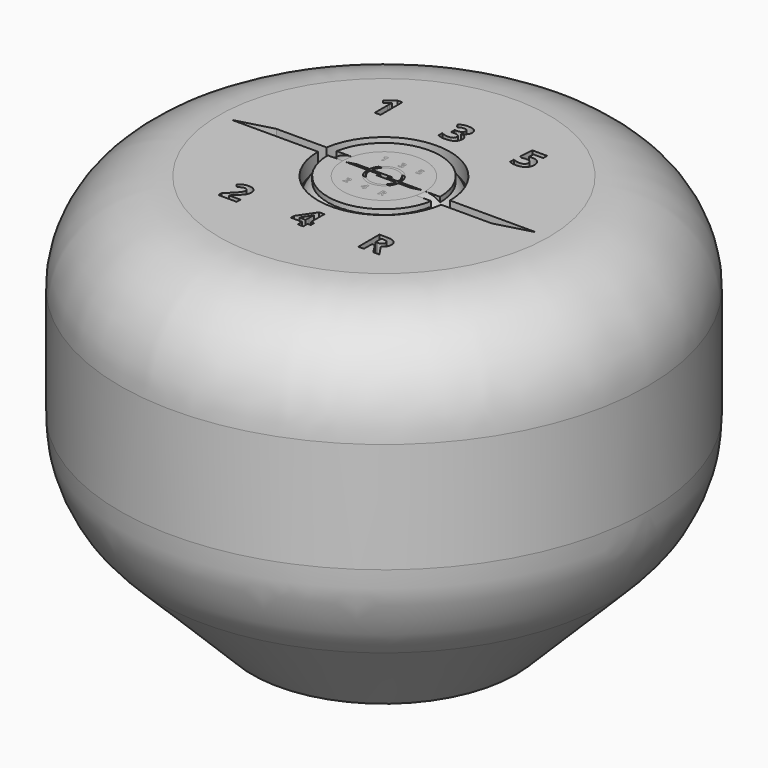
from build123d import *

# Parameters (mm, degrees)
F1_R           = 101.6
F2_DEPTH       = 152.4
F3_R           = 38.1
F4_SIZE        = 50.8
F5_R           = 50.8
F6_TEXT_SIZE   = 14.6624815095
F6_TEXT_SIZE_2 = 14.2217245241
F7_DEPTH       = 6.35
F8_SCALE       = 0.25


# Not quite as in the source:
# - Text() gives the source's letters only with a copy of the font that has no kerning and outlines rounded to 1/6400 em; it was checked with that copy


with BuildPart() as f2:
    # F1 (on Top) → F2 (new body)
    with BuildSketch(Plane.XY):
        Circle(F1_R)
    extrude(amount=-F2_DEPTH)

    # F3
    f3_edges = [f2.edges().sort_by_distance(p)[0] for p in [
        (-101.6, 0, 0),
    ]]
    fillet(f3_edges, radius=F3_R)

    # F4
    f4_edges = [f2.edges().sort_by_distance(p)[0] for p in [
        (-101.6, 0, -152.4),
    ]]
    chamfer(f4_edges, length=F4_SIZE)

    # F5
    f5_edges = [f2.edges().sort_by_distance(p)[0] for p in [
        (-101.6, 0, -101.6),
    ]]
    fillet(f5_edges, radius=F5_R)

    # F0 (on Top) + F6 (on Top) → F7 (cut)
    with BuildSketch(Plane.XY):
        with BuildLine():
            Line((-25.1126263436, 3.81), (-44.4500020284, 3.81))
            Line((-44.4500020284, 3.81), (-58.4200020284, 0))
            Line((-58.4200020284, 0), (-25.4000020284, 0))
            ThreePointArc((-25.4000020284, 0), (-1.9104132919, -25.3280541851), (25.1126222869, -3.81))
            Line((25.1126222869, -3.81), (44.4499979716, -3.81))
            Line((44.4499979716, -3.81), (58.4199979716, 0))
            Line((58.4199979716, 0), (25.3999979716, 0))
            ThreePointArc((25.3999979716, 0), (1.9104092352, 25.3280541851), (-25.1126263436, 3.81))
        make_face()
        with BuildLine():
            Line((-5.0800020284, 0), (-10.1600020284, -3.81))
            Line((-10.1600020284, -3.81), (21.2511626456, -3.81))
            ThreePointArc((21.2511626456, -3.81), (-1.9125206151, -21.5051243348), (-21.5900020284, 0))
            Line((-21.5900020284, 0), (-5.0800020284, 0))
        make_face(mode=Mode.SUBTRACT)
        with BuildLine():
            Line((5.0799979716, 0), (10.1599979716, 3.81))
            Line((10.1599979716, 3.81), (-21.2511667023, 3.81))
            ThreePointArc((-21.2511667023, 3.81), (1.9125165584, 21.5051243348), (21.5899979716, 0))
            Line((21.5899979716, 0), (5.0799979716, 0))
        make_face(mode=Mode.SUBTRACT)
    with BuildSketch(Plane.XY):
        with Locations((-31.75, 30.48)):
            Text('1     3     5', F6_TEXT_SIZE, font='Open Sans', font_style=FontStyle.BOLD, text_align=(TextAlign.LEFT, TextAlign.BOTTOM))
        with Locations((-31.75, -40.7196416573)):
            Text('2     4     R', F6_TEXT_SIZE_2, font='Open Sans', font_style=FontStyle.BOLD, text_align=(TextAlign.LEFT, TextAlign.BOTTOM))
    extrude(amount=-F7_DEPTH, mode=Mode.SUBTRACT)


with BuildPart() as f8_1:
    # F8: copy of F2
    add(f2.part.scale(F8_SCALE))


solid = Compound([f2.part, f8_1.part])
